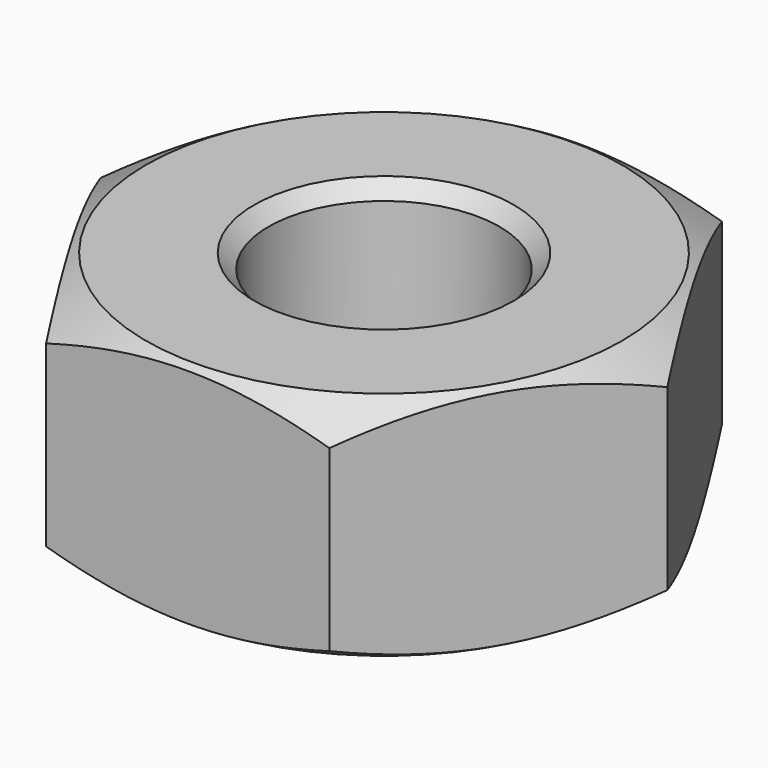
from build123d import *

# Parameters (mm, degrees)
F0_R     = 4
F1_DEPTH = 8
F4_SIZE  = 0.5


# Not quite as in the source:
# - a feature of the source that left no trace in its solid (it failed there, or was rolled back) is left out


with BuildPart() as f1:
    # F0 (on Top) → F1 (new body)
    with BuildSketch(Plane.XY):
        Polygon((4.9074772881, -8.5), (9.8149545762, 0), (4.9074772881, 8.5), (-4.9074772881, 8.5), (-9.8149545762, 0), (-4.9074772881, -8.5), align=None)
        Circle(F0_R, mode=Mode.SUBTRACT)
    extrude(amount=F1_DEPTH)

    # F2 (on Front) → F3 (revolve, cut)
    with BuildSketch(Plane.XZ):
        Polygon((12.4901464933, 8), (8.25, 8), (12.4901464933, 5.5519502807), align=None)
        Polygon((12.4901464933, 2.4480497193), (8.25, 0), (12.4901464933, 0), align=None)
    revolve(axis=Axis((0, 0, 3.4472336993), (0, 0, -1)), mode=Mode.SUBTRACT)

    # F4
    f4_edges = [f1.edges().sort_by_distance(p)[0] for p in [
        (-4, 0, 8),
        (-4, 0, 0),
    ]]
    chamfer(f4_edges, length=F4_SIZE)


solid = f1.part
